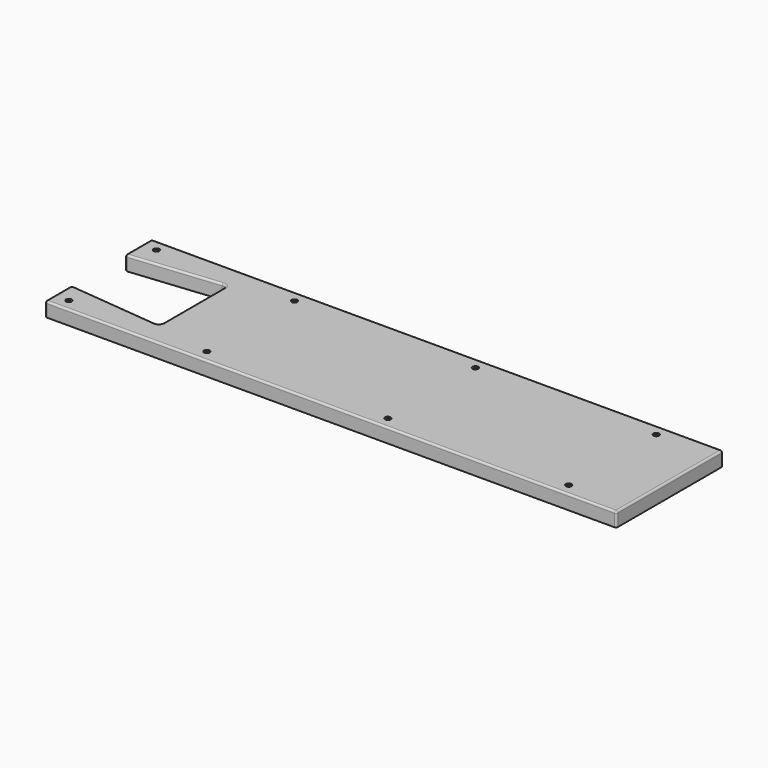
from build123d import *

# Parameters (mm, degrees)
F1_DEPTH       = 7.5
F3_DEPTH       = 10
F5_D           = 4
F5_CSINK_D     = 6
F5_CSINK_ANGLE = 90
F6_R           = 2


# Not quite as in the source:
# - a feature names something its author has since deleted; it is built from what else it names


with BuildPart() as f1:
    # F0 (on Top) → F1 (new body, symmetric)
    with BuildSketch(Plane.XY):
        with BuildLine():
            Line((-300, -70), (300, -70))
            Line((300, -70), (300, 70))
            Line((300, 70), (-300, 70))
            Line((-300, 70), (-300, 35))
            Line((-300, 35), (-205.4975185951, 44.4502481405))
            ThreePointArc((-205.4975185951, 44.4502481405), (-201.6449733962, 43.1823248572), (-200, 39.4750621894))
            Line((-200, 39.4750621894), (-200, 0))
            Line((-200, 0), (-200, -39.4750621894))
            ThreePointArc((-200, -39.4750621894), (-201.6449733962, -43.1823248572), (-205.4975185951, -44.4502481405))
            Line((-205.4975185951, -44.4502481405), (-300, -35))
            Line((-300, -35), (-300, -70))
        make_face()
    extrude(amount=F1_DEPTH, both=True)

    # F2 (on face) → F3 (cut)
    with BuildSketch(Plane(origin=(0, 0, -7.5), x_dir=(1, 0, 0), z_dir=(0, 0, -1))):
        with BuildLine():
            Line((-175, 40), (-175, 0))
            Line((-175, 0), (-175, -40))
            ThreePointArc((-175, -40), (-173.5355339059, -43.5355339059), (-170, -45))
            Line((-170, -45), (270, -45))
            ThreePointArc((270, -45), (273.5355339059, -43.5355339059), (275, -40))
            Line((275, -40), (275, 0))
            Line((275, 0), (275, 40))
            ThreePointArc((275, 40), (273.5355339059, 43.5355339059), (270, 45))
            Line((270, 45), (-170, 45))
            ThreePointArc((-170, 45), (-173.5355339059, 43.5355339059), (-175, 40))
        make_face()
    extrude(amount=-F3_DEPTH, mode=Mode.SUBTRACT)

    # F5 (through all)
    with Locations(Plane.XY.offset(7.5)):
        with Locations((-285, 57.5), (-285, -57.5), (-140, -57.5), (50, -57.5), (240, -57.5), (240, 57.5), (50, 57.5), (-140, 57.5)):
            CounterSinkHole(F5_D / 2, F5_CSINK_D / 2, counter_sink_angle=F5_CSINK_ANGLE)

    # F6
    f6_edges = [f1.edges().sort_by_distance(p)[0] for p in [
        (0, -70, 7.5),
        (-300, -52.5, 7.5),
        (-252.748759, -39.725124, 7.5),
        (0, 70, 7.5),
        (-300, 52.5, 7.5),
        (300, 0, 7.5),
        (-175, 0, -7.5),
        (-300, 35, 0),
        (-300, -70, 0),
        (-300, 70, 0),
        (300, 70, 0),
        (300, -70, 0),
        (-300, -35, 0),
    ]]
    fillet(f6_edges, radius=F6_R)


solid = f1.part
